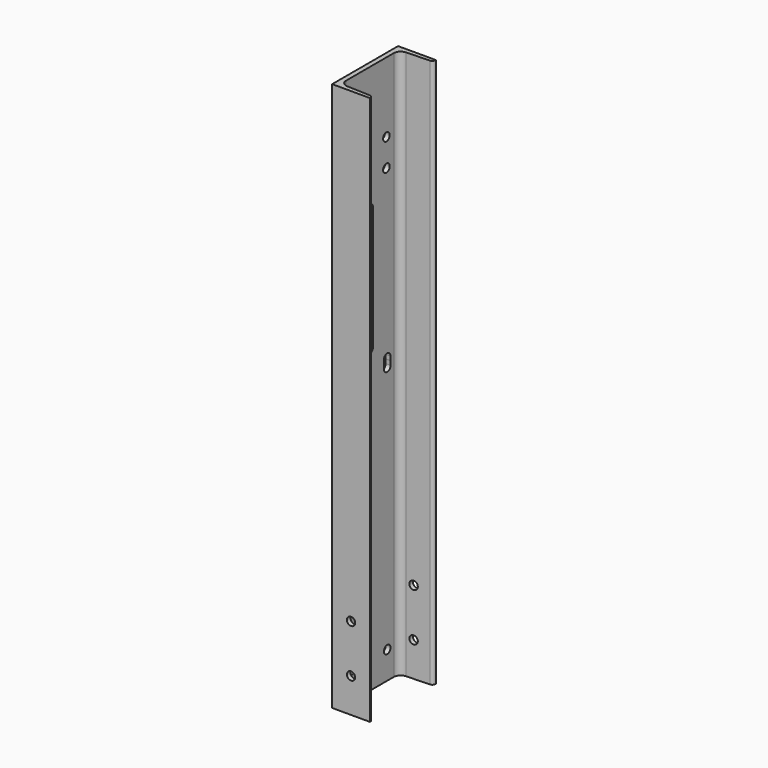
from build123d import *

# Parameters (mm, degrees)
F1_DEPTH = 400
F2_R     = 6
F3_DEPTH = 55.001
F4_R     = 6
F5_DEPTH = 120.001


# Not quite as in the source:
# - a feature names something its author has since deleted; it is built from what else it names


with BuildPart() as f1:
    # F0 (on Top) → F1 (new body, symmetric)
    with BuildSketch(Plane.XY):
        with BuildLine():
            Line((0, 120), (0, 0))
            Line((0, 0), (55, 0))
            Line((55, 0), (55, 0.683595444))
            ThreePointArc((55, 0.683595444), (53.7475389551, 3.7986380977), (50.6873374512, 5.1796942729))
            Line((50.6873374512, 5.1796942729), (16.5836945529, 6.6006793936))
            ThreePointArc((16.5836945529, 6.6006793936), (9.7832467663, 9.6696931162), (7, 16.5920101246))
            Line((7, 16.5920101246), (7, 103.4079898754))
            ThreePointArc((7, 103.4079898754), (9.7832467663, 110.3303068838), (16.5836945529, 113.3993206064))
            Line((16.5836945529, 113.3993206064), (50.6873374512, 114.8203057271))
            ThreePointArc((50.6873374512, 114.8203057271), (53.7475389551, 116.2013619023), (55, 119.316404556))
            Line((55, 119.316404556), (55, 120))
            Line((55, 120), (0, 120))
        make_face()
    extrude(amount=F1_DEPTH, both=True)

    # F2 (on face) → F3 (cut, through all)
    with BuildSketch(Plane(origin=(0, 0, 0), x_dir=(0, -1, 0), z_dir=(-1, 0, 0))):
        with Locations((-90, 298)):
            Circle(F2_R)
        with Locations((-30, 298)):
            Circle(F2_R)
        with Locations((-30, 258)):
            Circle(F2_R)
        with Locations((-90, 258)):
            Circle(F2_R)
        with BuildLine():
            Line((-97.4973066239, 7.8202411081), (-97.4971376848, 8.1853094437))
            ThreePointArc((-97.4971376848, 8.1853094437), (-97.4999993576, 8.0027765611), (-97.4973066239, 7.8202411081))
        make_face()
        with Locations((-91.5, -360)):
            Circle(F2_R)
        with Locations((-28.5, -360)):
            Circle(F2_R)
        with BuildLine():
            Line((-97.4945650308, 13.7446764959), (-97.4971376848, 8.1853094437))
            Line((-97.4971376848, 8.1853094437), (-97.4973066239, 7.8202411081))
            Line((-97.4973066239, 7.8202411081), (-97.4999974302, 2.0055531216))
            ThreePointArc((-97.4999974302, 2.0055531216), (-97.4999993576, 2.0027765611), (-97.5, 2))
            ThreePointArc((-97.5, 2), (-91.5, -4), (-85.5, 2))
            Line((-85.5, 2), (-85.5, 14))
            ThreePointArc((-85.5, 14), (-91.6276906718, 19.9986411038), (-97.4945650308, 13.7446764959))
        make_face()
        with BuildLine():
            Line((-22.5, 2), (-22.5, 14))
            ThreePointArc((-22.5, 14), (-28.5, 20), (-34.5, 14))
            Line((-34.5, 14), (-34.5, 2))
            ThreePointArc((-34.5, 2), (-28.5, -4), (-22.5, 2))
        make_face()
        with BuildLine():
            Line((-65.5, 218), (-65.5, 38))
            ThreePointArc((-65.5, 38), (-60, 32.5), (-54.5, 38))
            Line((-54.5, 38), (-54.5, 218))
            ThreePointArc((-54.5, 218), (-60, 223.5), (-65.5, 218))
        make_face()
    extrude(amount=-F3_DEPTH, mode=Mode.SUBTRACT)

    # F4 (on face) → F5 (cut, through all)
    with BuildSketch(Plane.XZ):
        with Locations((27.5, -280)):
            Circle(F4_R)
        with Locations((27.5, -350)):
            Circle(F4_R)
    extrude(amount=-F5_DEPTH, mode=Mode.SUBTRACT)


solid = f1.part
